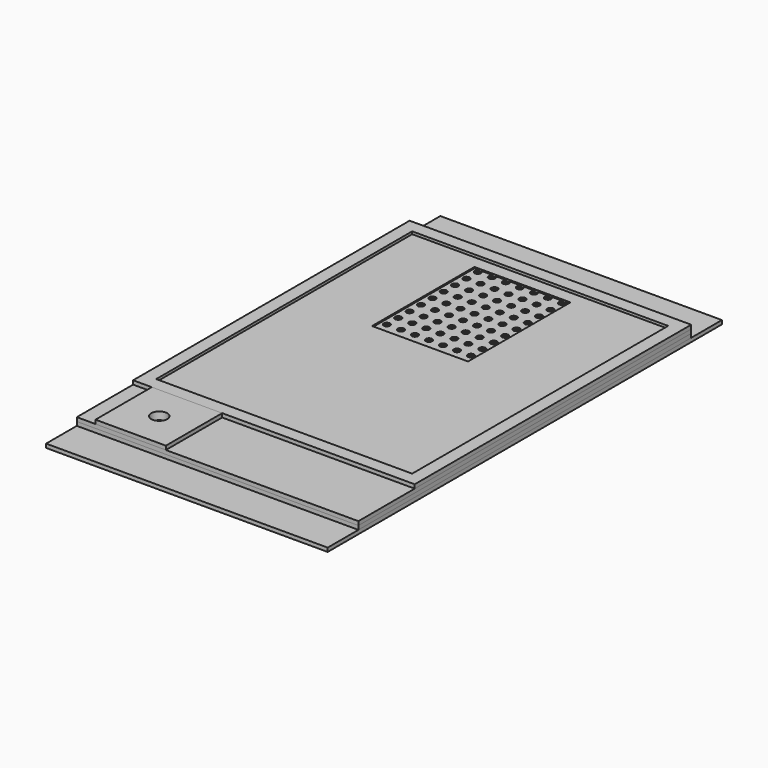
from build123d import *

# Parameters (mm, degrees)
F0_W      = 220
F0_H      = 270
F0_W_2    = 200
F0_H_2    = 250
F1_DEPTH  = 3
F2_W      = 220
F2_H      = 325
F2_R      = 17.07
F2_R_2    = 2.5
F3_DEPTH  = 3
F4_W      = 220
F4_H      = 325
F4_R      = 17.07
F4_R_2    = 1
F5_DEPTH  = 3
F6_W      = 220
F6_H      = 325
F6_W_2    = 90
F6_H_2    = 65
F6_W_3    = 70.7
F6_H_3    = 5.5
F7_DEPTH  = 3
F8_W      = 220
F8_H      = 385
F9_DEPTH  = 3
F10_DEPTH = 3
F11_W     = 55
F11_H     = 55
F12_DEPTH = 3
F13_R     = 6.25
F14_DEPTH = 12.001
F15_W     = 200
F15_H     = 250
F15_W_2   = 75
F15_H_2   = 100
F16_DEPTH = 1
F18_DEPTH = 1


with BuildPart() as f1:
    # F0 (on Top) → F1 (new body)
    with BuildSketch(Plane.XY):
        with Locations((100, 125)):
            Rectangle(F0_W, F0_H)
        with Locations((100, 125)):
            Rectangle(F0_W_2, F0_H_2, mode=Mode.SUBTRACT)
    extrude(amount=F1_DEPTH)


with BuildPart() as f3:
    # F2 (on Top) → F3 (new body)
    with BuildSketch(Plane.XY):
        with Locations((100, 97.5)):
            Rectangle(F2_W, F2_H)
        with Locations((32.07, -37.07)):
            Circle(F2_R, mode=Mode.SUBTRACT)
        with Locations((17.5, 15.5)):
            Circle(F2_R_2, mode=Mode.SUBTRACT)
        with Locations((28.45, 15.5)):
            Circle(F2_R_2, mode=Mode.SUBTRACT)
        with Locations((39.4, 15.5)):
            Circle(F2_R_2, mode=Mode.SUBTRACT)
        with Locations((50.35, 15.5)):
            Circle(F2_R_2, mode=Mode.SUBTRACT)
        with Locations((61.3, 15.5)):
            Circle(F2_R_2, mode=Mode.SUBTRACT)
        with Locations((72.25, 15.5)):
            Circle(F2_R_2, mode=Mode.SUBTRACT)
        with Locations((83.2, 15.5)):
            Circle(F2_R_2, mode=Mode.SUBTRACT)
        with Locations((94.15, 15.5)):
            Circle(F2_R_2, mode=Mode.SUBTRACT)
        with Locations((17.5, 26.6)):
            Circle(F2_R_2, mode=Mode.SUBTRACT)
        with Locations((28.45, 26.6)):
            Circle(F2_R_2, mode=Mode.SUBTRACT)
        with Locations((39.4, 26.6)):
            Circle(F2_R_2, mode=Mode.SUBTRACT)
        with Locations((17.5, 37.7)):
            Circle(F2_R_2, mode=Mode.SUBTRACT)
        with Locations((28.45, 37.7)):
            Circle(F2_R_2, mode=Mode.SUBTRACT)
        with Locations((17.5, 48.8)):
            Circle(F2_R_2, mode=Mode.SUBTRACT)
        with Locations((28.45, 48.8)):
            Circle(F2_R_2, mode=Mode.SUBTRACT)
        with Locations((39.4, 37.7)):
            Circle(F2_R_2, mode=Mode.SUBTRACT)
        with Locations((39.4, 48.8)):
            Circle(F2_R_2, mode=Mode.SUBTRACT)
        with Locations((17.5, 59.9)):
            Circle(F2_R_2, mode=Mode.SUBTRACT)
        with Locations((28.45, 59.9)):
            Circle(F2_R_2, mode=Mode.SUBTRACT)
        with Locations((17.5, 71)):
            Circle(F2_R_2, mode=Mode.SUBTRACT)
        with Locations((28.45, 71)):
            Circle(F2_R_2, mode=Mode.SUBTRACT)
        with Locations((39.4, 59.9)):
            Circle(F2_R_2, mode=Mode.SUBTRACT)
        with Locations((39.4, 71)):
            Circle(F2_R_2, mode=Mode.SUBTRACT)
        with Locations((17.5, 82.1)):
            Circle(F2_R_2, mode=Mode.SUBTRACT)
        with Locations((28.45, 82.1)):
            Circle(F2_R_2, mode=Mode.SUBTRACT)
        with Locations((17.5, 93.2)):
            Circle(F2_R_2, mode=Mode.SUBTRACT)
        with Locations((28.45, 93.2)):
            Circle(F2_R_2, mode=Mode.SUBTRACT)
        with Locations((39.4, 82.1)):
            Circle(F2_R_2, mode=Mode.SUBTRACT)
        with Locations((39.4, 93.2)):
            Circle(F2_R_2, mode=Mode.SUBTRACT)
        with Locations((50.35, 26.6)):
            Circle(F2_R_2, mode=Mode.SUBTRACT)
        with Locations((61.3, 26.6)):
            Circle(F2_R_2, mode=Mode.SUBTRACT)
        with Locations((72.25, 26.6)):
            Circle(F2_R_2, mode=Mode.SUBTRACT)
        with Locations((50.35, 37.7)):
            Circle(F2_R_2, mode=Mode.SUBTRACT)
        with Locations((50.35, 48.8)):
            Circle(F2_R_2, mode=Mode.SUBTRACT)
        with Locations((61.3, 37.7)):
            Circle(F2_R_2, mode=Mode.SUBTRACT)
        with Locations((72.25, 37.7)):
            Circle(F2_R_2, mode=Mode.SUBTRACT)
        with Locations((61.3, 48.8)):
            Circle(F2_R_2, mode=Mode.SUBTRACT)
        with Locations((72.25, 48.8)):
            Circle(F2_R_2, mode=Mode.SUBTRACT)
        with Locations((83.2, 26.6)):
            Circle(F2_R_2, mode=Mode.SUBTRACT)
        with Locations((94.15, 26.6)):
            Circle(F2_R_2, mode=Mode.SUBTRACT)
        with Locations((83.2, 37.7)):
            Circle(F2_R_2, mode=Mode.SUBTRACT)
        with Locations((83.2, 48.8)):
            Circle(F2_R_2, mode=Mode.SUBTRACT)
        with Locations((94.15, 37.7)):
            Circle(F2_R_2, mode=Mode.SUBTRACT)
        with Locations((94.15, 48.8)):
            Circle(F2_R_2, mode=Mode.SUBTRACT)
        with Locations((50.35, 59.9)):
            Circle(F2_R_2, mode=Mode.SUBTRACT)
        with Locations((50.35, 71)):
            Circle(F2_R_2, mode=Mode.SUBTRACT)
        with Locations((61.3, 59.9)):
            Circle(F2_R_2, mode=Mode.SUBTRACT)
        with Locations((72.25, 59.9)):
            Circle(F2_R_2, mode=Mode.SUBTRACT)
        with Locations((61.3, 71)):
            Circle(F2_R_2, mode=Mode.SUBTRACT)
        with Locations((72.25, 71)):
            Circle(F2_R_2, mode=Mode.SUBTRACT)
        with Locations((50.35, 82.1)):
            Circle(F2_R_2, mode=Mode.SUBTRACT)
        with Locations((50.35, 93.2)):
            Circle(F2_R_2, mode=Mode.SUBTRACT)
        with Locations((61.3, 82.1)):
            Circle(F2_R_2, mode=Mode.SUBTRACT)
        with Locations((72.25, 82.1)):
            Circle(F2_R_2, mode=Mode.SUBTRACT)
        with Locations((61.3, 93.2)):
            Circle(F2_R_2, mode=Mode.SUBTRACT)
        with Locations((72.25, 93.2)):
            Circle(F2_R_2, mode=Mode.SUBTRACT)
        with Locations((83.2, 59.9)):
            Circle(F2_R_2, mode=Mode.SUBTRACT)
        with Locations((83.2, 71)):
            Circle(F2_R_2, mode=Mode.SUBTRACT)
        with Locations((94.15, 59.9)):
            Circle(F2_R_2, mode=Mode.SUBTRACT)
        with Locations((94.15, 71)):
            Circle(F2_R_2, mode=Mode.SUBTRACT)
        with Locations((83.2, 82.1)):
            Circle(F2_R_2, mode=Mode.SUBTRACT)
        with Locations((83.2, 93.2)):
            Circle(F2_R_2, mode=Mode.SUBTRACT)
        with Locations((94.15, 82.1)):
            Circle(F2_R_2, mode=Mode.SUBTRACT)
        with Locations((94.15, 93.2)):
            Circle(F2_R_2, mode=Mode.SUBTRACT)
        with Locations((105.1, 15.5)):
            Circle(F2_R_2, mode=Mode.SUBTRACT)
        with Locations((116.05, 15.5)):
            Circle(F2_R_2, mode=Mode.SUBTRACT)
        with Locations((127, 15.5)):
            Circle(F2_R_2, mode=Mode.SUBTRACT)
        with Locations((137.95, 15.5)):
            Circle(F2_R_2, mode=Mode.SUBTRACT)
        with Locations((148.9, 15.5)):
            Circle(F2_R_2, mode=Mode.SUBTRACT)
        with Locations((159.85, 15.5)):
            Circle(F2_R_2, mode=Mode.SUBTRACT)
        with Locations((170.8, 15.5)):
            Circle(F2_R_2, mode=Mode.SUBTRACT)
        with Locations((181.75, 15.5)):
            Circle(F2_R_2, mode=Mode.SUBTRACT)
        with Locations((105.1, 26.6)):
            Circle(F2_R_2, mode=Mode.SUBTRACT)
        with Locations((116.05, 26.6)):
            Circle(F2_R_2, mode=Mode.SUBTRACT)
        with Locations((127, 26.6)):
            Circle(F2_R_2, mode=Mode.SUBTRACT)
        with Locations((105.1, 37.7)):
            Circle(F2_R_2, mode=Mode.SUBTRACT)
        with Locations((105.1, 48.8)):
            Circle(F2_R_2, mode=Mode.SUBTRACT)
        with Locations((116.05, 37.7)):
            Circle(F2_R_2, mode=Mode.SUBTRACT)
        with Locations((127, 37.7)):
            Circle(F2_R_2, mode=Mode.SUBTRACT)
        with Locations((116.05, 48.8)):
            Circle(F2_R_2, mode=Mode.SUBTRACT)
        with Locations((127, 48.8)):
            Circle(F2_R_2, mode=Mode.SUBTRACT)
        with Locations((137.95, 26.6)):
            Circle(F2_R_2, mode=Mode.SUBTRACT)
        with Locations((148.9, 26.6)):
            Circle(F2_R_2, mode=Mode.SUBTRACT)
        with Locations((137.95, 37.7)):
            Circle(F2_R_2, mode=Mode.SUBTRACT)
        with Locations((137.95, 48.8)):
            Circle(F2_R_2, mode=Mode.SUBTRACT)
        with Locations((148.9, 37.7)):
            Circle(F2_R_2, mode=Mode.SUBTRACT)
        with Locations((148.9, 48.8)):
            Circle(F2_R_2, mode=Mode.SUBTRACT)
        with Locations((105.1, 59.9)):
            Circle(F2_R_2, mode=Mode.SUBTRACT)
        with Locations((105.1, 71)):
            Circle(F2_R_2, mode=Mode.SUBTRACT)
        with Locations((116.05, 59.9)):
            Circle(F2_R_2, mode=Mode.SUBTRACT)
        with Locations((127, 59.9)):
            Circle(F2_R_2, mode=Mode.SUBTRACT)
        with Locations((116.05, 71)):
            Circle(F2_R_2, mode=Mode.SUBTRACT)
        with Locations((127, 71)):
            Circle(F2_R_2, mode=Mode.SUBTRACT)
        with Locations((105.1, 82.1)):
            Circle(F2_R_2, mode=Mode.SUBTRACT)
        with Locations((105.1, 93.2)):
            Circle(F2_R_2, mode=Mode.SUBTRACT)
        with Locations((116.05, 82.1)):
            Circle(F2_R_2, mode=Mode.SUBTRACT)
        with Locations((127, 82.1)):
            Circle(F2_R_2, mode=Mode.SUBTRACT)
        with Locations((116.05, 93.2)):
            Circle(F2_R_2, mode=Mode.SUBTRACT)
        with Locations((127, 93.2)):
            Circle(F2_R_2, mode=Mode.SUBTRACT)
        with Locations((137.95, 59.9)):
            Circle(F2_R_2, mode=Mode.SUBTRACT)
        with Locations((137.95, 71)):
            Circle(F2_R_2, mode=Mode.SUBTRACT)
        with Locations((148.9, 59.9)):
            Circle(F2_R_2, mode=Mode.SUBTRACT)
        with Locations((148.9, 71)):
            Circle(F2_R_2, mode=Mode.SUBTRACT)
        with Locations((137.95, 82.1)):
            Circle(F2_R_2, mode=Mode.SUBTRACT)
        with Locations((137.95, 93.2)):
            Circle(F2_R_2, mode=Mode.SUBTRACT)
        with Locations((148.9, 82.1)):
            Circle(F2_R_2, mode=Mode.SUBTRACT)
        with Locations((148.9, 93.2)):
            Circle(F2_R_2, mode=Mode.SUBTRACT)
        with Locations((159.85, 26.6)):
            Circle(F2_R_2, mode=Mode.SUBTRACT)
        with Locations((170.8, 26.6)):
            Circle(F2_R_2, mode=Mode.SUBTRACT)
        with Locations((181.75, 26.6)):
            Circle(F2_R_2, mode=Mode.SUBTRACT)
        with Locations((159.85, 37.7)):
            Circle(F2_R_2, mode=Mode.SUBTRACT)
        with Locations((159.85, 48.8)):
            Circle(F2_R_2, mode=Mode.SUBTRACT)
        with Locations((170.8, 37.7)):
            Circle(F2_R_2, mode=Mode.SUBTRACT)
        with Locations((181.75, 37.7)):
            Circle(F2_R_2, mode=Mode.SUBTRACT)
        with Locations((170.8, 48.8)):
            Circle(F2_R_2, mode=Mode.SUBTRACT)
        with Locations((181.75, 48.8)):
            Circle(F2_R_2, mode=Mode.SUBTRACT)
        with Locations((159.85, 59.9)):
            Circle(F2_R_2, mode=Mode.SUBTRACT)
        with Locations((159.85, 71)):
            Circle(F2_R_2, mode=Mode.SUBTRACT)
        with Locations((170.8, 59.9)):
            Circle(F2_R_2, mode=Mode.SUBTRACT)
        with Locations((181.75, 59.9)):
            Circle(F2_R_2, mode=Mode.SUBTRACT)
        with Locations((170.8, 71)):
            Circle(F2_R_2, mode=Mode.SUBTRACT)
        with Locations((181.75, 71)):
            Circle(F2_R_2, mode=Mode.SUBTRACT)
        with Locations((159.85, 82.1)):
            Circle(F2_R_2, mode=Mode.SUBTRACT)
        with Locations((159.85, 93.2)):
            Circle(F2_R_2, mode=Mode.SUBTRACT)
        with Locations((170.8, 82.1)):
            Circle(F2_R_2, mode=Mode.SUBTRACT)
        with Locations((181.75, 82.1)):
            Circle(F2_R_2, mode=Mode.SUBTRACT)
        with Locations((170.8, 93.2)):
            Circle(F2_R_2, mode=Mode.SUBTRACT)
        with Locations((181.75, 93.2)):
            Circle(F2_R_2, mode=Mode.SUBTRACT)
        with Locations((17.5, 104.3)):
            Circle(F2_R_2, mode=Mode.SUBTRACT)
        with Locations((28.45, 104.3)):
            Circle(F2_R_2, mode=Mode.SUBTRACT)
        with Locations((17.5, 115.4)):
            Circle(F2_R_2, mode=Mode.SUBTRACT)
        with Locations((28.45, 115.4)):
            Circle(F2_R_2, mode=Mode.SUBTRACT)
        with Locations((39.4, 104.3)):
            Circle(F2_R_2, mode=Mode.SUBTRACT)
        with Locations((39.4, 115.4)):
            Circle(F2_R_2, mode=Mode.SUBTRACT)
        with Locations((17.5, 126.5)):
            Circle(F2_R_2, mode=Mode.SUBTRACT)
        with Locations((28.45, 126.5)):
            Circle(F2_R_2, mode=Mode.SUBTRACT)
        with Locations((17.5, 137.6)):
            Circle(F2_R_2, mode=Mode.SUBTRACT)
        with Locations((28.45, 137.6)):
            Circle(F2_R_2, mode=Mode.SUBTRACT)
        with Locations((39.4, 126.5)):
            Circle(F2_R_2, mode=Mode.SUBTRACT)
        with Locations((39.4, 137.6)):
            Circle(F2_R_2, mode=Mode.SUBTRACT)
        with Locations((17.5, 148.7)):
            Circle(F2_R_2, mode=Mode.SUBTRACT)
        with Locations((28.45, 148.7)):
            Circle(F2_R_2, mode=Mode.SUBTRACT)
        with Locations((39.4, 148.7)):
            Circle(F2_R_2, mode=Mode.SUBTRACT)
        with Locations((17.5, 159.8)):
            Circle(F2_R_2, mode=Mode.SUBTRACT)
        with Locations((28.45, 159.8)):
            Circle(F2_R_2, mode=Mode.SUBTRACT)
        with Locations((17.5, 170.9)):
            Circle(F2_R_2, mode=Mode.SUBTRACT)
        with Locations((28.45, 170.9)):
            Circle(F2_R_2, mode=Mode.SUBTRACT)
        with Locations((39.4, 159.8)):
            Circle(F2_R_2, mode=Mode.SUBTRACT)
        with Locations((39.4, 170.9)):
            Circle(F2_R_2, mode=Mode.SUBTRACT)
        with Locations((50.35, 104.3)):
            Circle(F2_R_2, mode=Mode.SUBTRACT)
        with Locations((50.35, 115.4)):
            Circle(F2_R_2, mode=Mode.SUBTRACT)
        with Locations((61.3, 104.3)):
            Circle(F2_R_2, mode=Mode.SUBTRACT)
        with Locations((72.25, 104.3)):
            Circle(F2_R_2, mode=Mode.SUBTRACT)
        with Locations((61.3, 115.4)):
            Circle(F2_R_2, mode=Mode.SUBTRACT)
        with Locations((72.25, 115.4)):
            Circle(F2_R_2, mode=Mode.SUBTRACT)
        with Locations((50.35, 126.5)):
            Circle(F2_R_2, mode=Mode.SUBTRACT)
        with Locations((50.35, 137.6)):
            Circle(F2_R_2, mode=Mode.SUBTRACT)
        with Locations((61.3, 126.5)):
            Circle(F2_R_2, mode=Mode.SUBTRACT)
        with Locations((72.25, 126.5)):
            Circle(F2_R_2, mode=Mode.SUBTRACT)
        with Locations((61.3, 137.6)):
            Circle(F2_R_2, mode=Mode.SUBTRACT)
        with Locations((72.25, 137.6)):
            Circle(F2_R_2, mode=Mode.SUBTRACT)
        with Locations((83.2, 104.3)):
            Circle(F2_R_2, mode=Mode.SUBTRACT)
        with Locations((83.2, 115.4)):
            Circle(F2_R_2, mode=Mode.SUBTRACT)
        with Locations((94.15, 104.3)):
            Circle(F2_R_2, mode=Mode.SUBTRACT)
        with Locations((94.15, 115.4)):
            Circle(F2_R_2, mode=Mode.SUBTRACT)
        with Locations((83.2, 126.5)):
            Circle(F2_R_2, mode=Mode.SUBTRACT)
        with Locations((83.2, 137.6)):
            Circle(F2_R_2, mode=Mode.SUBTRACT)
        with Locations((94.15, 126.5)):
            Circle(F2_R_2, mode=Mode.SUBTRACT)
        with Locations((94.15, 137.6)):
            Circle(F2_R_2, mode=Mode.SUBTRACT)
        with Locations((50.35, 148.7)):
            Circle(F2_R_2, mode=Mode.SUBTRACT)
        with Locations((61.3, 148.7)):
            Circle(F2_R_2, mode=Mode.SUBTRACT)
        with Locations((72.25, 148.7)):
            Circle(F2_R_2, mode=Mode.SUBTRACT)
        with Locations((50.35, 159.8)):
            Circle(F2_R_2, mode=Mode.SUBTRACT)
        with Locations((50.35, 170.9)):
            Circle(F2_R_2, mode=Mode.SUBTRACT)
        with Locations((61.3, 159.8)):
            Circle(F2_R_2, mode=Mode.SUBTRACT)
        with Locations((72.25, 159.8)):
            Circle(F2_R_2, mode=Mode.SUBTRACT)
        with Locations((61.3, 170.9)):
            Circle(F2_R_2, mode=Mode.SUBTRACT)
        with Locations((72.25, 170.9)):
            Circle(F2_R_2, mode=Mode.SUBTRACT)
        with Locations((83.2, 148.7)):
            Circle(F2_R_2, mode=Mode.SUBTRACT)
        with Locations((94.15, 148.7)):
            Circle(F2_R_2, mode=Mode.SUBTRACT)
        with Locations((83.2, 159.8)):
            Circle(F2_R_2, mode=Mode.SUBTRACT)
        with Locations((83.2, 170.9)):
            Circle(F2_R_2, mode=Mode.SUBTRACT)
        with Locations((94.15, 159.8)):
            Circle(F2_R_2, mode=Mode.SUBTRACT)
        with Locations((94.15, 170.9)):
            Circle(F2_R_2, mode=Mode.SUBTRACT)
        with Locations((17.5, 182)):
            Circle(F2_R_2, mode=Mode.SUBTRACT)
        with Locations((28.45, 182)):
            Circle(F2_R_2, mode=Mode.SUBTRACT)
        with Locations((17.5, 193.1)):
            Circle(F2_R_2, mode=Mode.SUBTRACT)
        with Locations((28.45, 193.1)):
            Circle(F2_R_2, mode=Mode.SUBTRACT)
        with Locations((39.4, 182)):
            Circle(F2_R_2, mode=Mode.SUBTRACT)
        with Locations((39.4, 193.1)):
            Circle(F2_R_2, mode=Mode.SUBTRACT)
        with Locations((17.5, 204.2)):
            Circle(F2_R_2, mode=Mode.SUBTRACT)
        with Locations((28.45, 204.2)):
            Circle(F2_R_2, mode=Mode.SUBTRACT)
        with Locations((17.5, 215.3)):
            Circle(F2_R_2, mode=Mode.SUBTRACT)
        with Locations((28.45, 215.3)):
            Circle(F2_R_2, mode=Mode.SUBTRACT)
        with Locations((39.4, 204.2)):
            Circle(F2_R_2, mode=Mode.SUBTRACT)
        with Locations((39.4, 215.3)):
            Circle(F2_R_2, mode=Mode.SUBTRACT)
        with Locations((17.5, 226.4)):
            Circle(F2_R_2, mode=Mode.SUBTRACT)
        with Locations((28.45, 226.4)):
            Circle(F2_R_2, mode=Mode.SUBTRACT)
        with Locations((17.5, 237.5)):
            Circle(F2_R_2, mode=Mode.SUBTRACT)
        with Locations((28.45, 237.5)):
            Circle(F2_R_2, mode=Mode.SUBTRACT)
        with Locations((39.4, 226.4)):
            Circle(F2_R_2, mode=Mode.SUBTRACT)
        with Locations((39.4, 237.5)):
            Circle(F2_R_2, mode=Mode.SUBTRACT)
        with Locations((50.35, 182)):
            Circle(F2_R_2, mode=Mode.SUBTRACT)
        with Locations((50.35, 193.1)):
            Circle(F2_R_2, mode=Mode.SUBTRACT)
        with Locations((61.3, 182)):
            Circle(F2_R_2, mode=Mode.SUBTRACT)
        with Locations((72.25, 182)):
            Circle(F2_R_2, mode=Mode.SUBTRACT)
        with Locations((61.3, 193.1)):
            Circle(F2_R_2, mode=Mode.SUBTRACT)
        with Locations((72.25, 193.1)):
            Circle(F2_R_2, mode=Mode.SUBTRACT)
        with Locations((50.35, 204.2)):
            Circle(F2_R_2, mode=Mode.SUBTRACT)
        with Locations((50.35, 215.3)):
            Circle(F2_R_2, mode=Mode.SUBTRACT)
        with Locations((61.3, 204.2)):
            Circle(F2_R_2, mode=Mode.SUBTRACT)
        with Locations((72.25, 204.2)):
            Circle(F2_R_2, mode=Mode.SUBTRACT)
        with Locations((61.3, 215.3)):
            Circle(F2_R_2, mode=Mode.SUBTRACT)
        with Locations((72.25, 215.3)):
            Circle(F2_R_2, mode=Mode.SUBTRACT)
        with Locations((83.2, 182)):
            Circle(F2_R_2, mode=Mode.SUBTRACT)
        with Locations((83.2, 193.1)):
            Circle(F2_R_2, mode=Mode.SUBTRACT)
        with Locations((94.15, 182)):
            Circle(F2_R_2, mode=Mode.SUBTRACT)
        with Locations((94.15, 193.1)):
            Circle(F2_R_2, mode=Mode.SUBTRACT)
        with Locations((83.2, 204.2)):
            Circle(F2_R_2, mode=Mode.SUBTRACT)
        with Locations((83.2, 215.3)):
            Circle(F2_R_2, mode=Mode.SUBTRACT)
        with Locations((94.15, 204.2)):
            Circle(F2_R_2, mode=Mode.SUBTRACT)
        with Locations((94.15, 215.3)):
            Circle(F2_R_2, mode=Mode.SUBTRACT)
        with Locations((50.35, 226.4)):
            Circle(F2_R_2, mode=Mode.SUBTRACT)
        with Locations((50.35, 237.5)):
            Circle(F2_R_2, mode=Mode.SUBTRACT)
        with Locations((61.3, 226.4)):
            Circle(F2_R_2, mode=Mode.SUBTRACT)
        with Locations((72.25, 226.4)):
            Circle(F2_R_2, mode=Mode.SUBTRACT)
        with Locations((61.3, 237.5)):
            Circle(F2_R_2, mode=Mode.SUBTRACT)
        with Locations((72.25, 237.5)):
            Circle(F2_R_2, mode=Mode.SUBTRACT)
        with Locations((83.2, 226.4)):
            Circle(F2_R_2, mode=Mode.SUBTRACT)
        with Locations((83.2, 237.5)):
            Circle(F2_R_2, mode=Mode.SUBTRACT)
        with Locations((94.15, 226.4)):
            Circle(F2_R_2, mode=Mode.SUBTRACT)
        with Locations((94.15, 237.5)):
            Circle(F2_R_2, mode=Mode.SUBTRACT)
        with Locations((105.1, 104.3)):
            Circle(F2_R_2, mode=Mode.SUBTRACT)
        with Locations((105.1, 115.4)):
            Circle(F2_R_2, mode=Mode.SUBTRACT)
        with Locations((116.05, 104.3)):
            Circle(F2_R_2, mode=Mode.SUBTRACT)
        with Locations((127, 104.3)):
            Circle(F2_R_2, mode=Mode.SUBTRACT)
        with Locations((116.05, 115.4)):
            Circle(F2_R_2, mode=Mode.SUBTRACT)
        with Locations((127, 115.4)):
            Circle(F2_R_2, mode=Mode.SUBTRACT)
        with Locations((105.1, 126.5)):
            Circle(F2_R_2, mode=Mode.SUBTRACT)
        with Locations((105.1, 137.6)):
            Circle(F2_R_2, mode=Mode.SUBTRACT)
        with Locations((116.05, 126.5)):
            Circle(F2_R_2, mode=Mode.SUBTRACT)
        with Locations((127, 126.5)):
            Circle(F2_R_2, mode=Mode.SUBTRACT)
        with Locations((116.05, 137.6)):
            Circle(F2_R_2, mode=Mode.SUBTRACT)
        with Locations((127, 137.6)):
            Circle(F2_R_2, mode=Mode.SUBTRACT)
        with Locations((137.95, 104.3)):
            Circle(F2_R_2, mode=Mode.SUBTRACT)
        with Locations((137.95, 115.4)):
            Circle(F2_R_2, mode=Mode.SUBTRACT)
        with Locations((148.9, 104.3)):
            Circle(F2_R_2, mode=Mode.SUBTRACT)
        with Locations((148.9, 115.4)):
            Circle(F2_R_2, mode=Mode.SUBTRACT)
        with Locations((137.95, 126.5)):
            Circle(F2_R_2, mode=Mode.SUBTRACT)
        with Locations((137.95, 137.6)):
            Circle(F2_R_2, mode=Mode.SUBTRACT)
        with Locations((148.9, 126.5)):
            Circle(F2_R_2, mode=Mode.SUBTRACT)
        with Locations((148.9, 137.6)):
            Circle(F2_R_2, mode=Mode.SUBTRACT)
        with Locations((105.1, 148.7)):
            Circle(F2_R_2, mode=Mode.SUBTRACT)
        with Locations((116.05, 148.7)):
            Circle(F2_R_2, mode=Mode.SUBTRACT)
        with Locations((127, 148.7)):
            Circle(F2_R_2, mode=Mode.SUBTRACT)
        with Locations((105.1, 159.8)):
            Circle(F2_R_2, mode=Mode.SUBTRACT)
        with Locations((105.1, 170.9)):
            Circle(F2_R_2, mode=Mode.SUBTRACT)
        with Locations((116.05, 159.8)):
            Circle(F2_R_2, mode=Mode.SUBTRACT)
        with Locations((127, 159.8)):
            Circle(F2_R_2, mode=Mode.SUBTRACT)
        with Locations((116.05, 170.9)):
            Circle(F2_R_2, mode=Mode.SUBTRACT)
        with Locations((127, 170.9)):
            Circle(F2_R_2, mode=Mode.SUBTRACT)
        with Locations((137.95, 148.7)):
            Circle(F2_R_2, mode=Mode.SUBTRACT)
        with Locations((148.9, 148.7)):
            Circle(F2_R_2, mode=Mode.SUBTRACT)
        with Locations((137.95, 159.8)):
            Circle(F2_R_2, mode=Mode.SUBTRACT)
        with Locations((137.95, 170.9)):
            Circle(F2_R_2, mode=Mode.SUBTRACT)
        with Locations((148.9, 159.8)):
            Circle(F2_R_2, mode=Mode.SUBTRACT)
        with Locations((148.9, 170.9)):
            Circle(F2_R_2, mode=Mode.SUBTRACT)
        with Locations((159.85, 104.3)):
            Circle(F2_R_2, mode=Mode.SUBTRACT)
        with Locations((159.85, 115.4)):
            Circle(F2_R_2, mode=Mode.SUBTRACT)
        with Locations((170.8, 104.3)):
            Circle(F2_R_2, mode=Mode.SUBTRACT)
        with Locations((181.75, 104.3)):
            Circle(F2_R_2, mode=Mode.SUBTRACT)
        with Locations((170.8, 115.4)):
            Circle(F2_R_2, mode=Mode.SUBTRACT)
        with Locations((181.75, 115.4)):
            Circle(F2_R_2, mode=Mode.SUBTRACT)
        with Locations((159.85, 126.5)):
            Circle(F2_R_2, mode=Mode.SUBTRACT)
        with Locations((159.85, 137.6)):
            Circle(F2_R_2, mode=Mode.SUBTRACT)
        with Locations((170.8, 126.5)):
            Circle(F2_R_2, mode=Mode.SUBTRACT)
        with Locations((181.75, 126.5)):
            Circle(F2_R_2, mode=Mode.SUBTRACT)
        with Locations((170.8, 137.6)):
            Circle(F2_R_2, mode=Mode.SUBTRACT)
        with Locations((181.75, 137.6)):
            Circle(F2_R_2, mode=Mode.SUBTRACT)
        with Locations((159.85, 148.7)):
            Circle(F2_R_2, mode=Mode.SUBTRACT)
        with Locations((170.8, 148.7)):
            Circle(F2_R_2, mode=Mode.SUBTRACT)
        with Locations((181.75, 148.7)):
            Circle(F2_R_2, mode=Mode.SUBTRACT)
        with Locations((159.85, 159.8)):
            Circle(F2_R_2, mode=Mode.SUBTRACT)
        with Locations((159.85, 170.9)):
            Circle(F2_R_2, mode=Mode.SUBTRACT)
        with Locations((170.8, 159.8)):
            Circle(F2_R_2, mode=Mode.SUBTRACT)
        with Locations((181.75, 159.8)):
            Circle(F2_R_2, mode=Mode.SUBTRACT)
        with Locations((170.8, 170.9)):
            Circle(F2_R_2, mode=Mode.SUBTRACT)
        with Locations((181.75, 170.9)):
            Circle(F2_R_2, mode=Mode.SUBTRACT)
        with Locations((105.1, 182)):
            Circle(F2_R_2, mode=Mode.SUBTRACT)
        with Locations((105.1, 193.1)):
            Circle(F2_R_2, mode=Mode.SUBTRACT)
        with Locations((116.05, 182)):
            Circle(F2_R_2, mode=Mode.SUBTRACT)
        with Locations((127, 182)):
            Circle(F2_R_2, mode=Mode.SUBTRACT)
        with Locations((116.05, 193.1)):
            Circle(F2_R_2, mode=Mode.SUBTRACT)
        with Locations((127, 193.1)):
            Circle(F2_R_2, mode=Mode.SUBTRACT)
        with Locations((105.1, 204.2)):
            Circle(F2_R_2, mode=Mode.SUBTRACT)
        with Locations((105.1, 215.3)):
            Circle(F2_R_2, mode=Mode.SUBTRACT)
        with Locations((116.05, 204.2)):
            Circle(F2_R_2, mode=Mode.SUBTRACT)
        with Locations((127, 204.2)):
            Circle(F2_R_2, mode=Mode.SUBTRACT)
        with Locations((116.05, 215.3)):
            Circle(F2_R_2, mode=Mode.SUBTRACT)
        with Locations((127, 215.3)):
            Circle(F2_R_2, mode=Mode.SUBTRACT)
        with Locations((137.95, 182)):
            Circle(F2_R_2, mode=Mode.SUBTRACT)
        with Locations((137.95, 193.1)):
            Circle(F2_R_2, mode=Mode.SUBTRACT)
        with Locations((148.9, 182)):
            Circle(F2_R_2, mode=Mode.SUBTRACT)
        with Locations((148.9, 193.1)):
            Circle(F2_R_2, mode=Mode.SUBTRACT)
        with Locations((137.95, 204.2)):
            Circle(F2_R_2, mode=Mode.SUBTRACT)
        with Locations((137.95, 215.3)):
            Circle(F2_R_2, mode=Mode.SUBTRACT)
        with Locations((148.9, 204.2)):
            Circle(F2_R_2, mode=Mode.SUBTRACT)
        with Locations((148.9, 215.3)):
            Circle(F2_R_2, mode=Mode.SUBTRACT)
        with Locations((105.1, 226.4)):
            Circle(F2_R_2, mode=Mode.SUBTRACT)
        with Locations((105.1, 237.5)):
            Circle(F2_R_2, mode=Mode.SUBTRACT)
        with Locations((116.05, 226.4)):
            Circle(F2_R_2, mode=Mode.SUBTRACT)
        with Locations((127, 226.4)):
            Circle(F2_R_2, mode=Mode.SUBTRACT)
        with Locations((116.05, 237.5)):
            Circle(F2_R_2, mode=Mode.SUBTRACT)
        with Locations((127, 237.5)):
            Circle(F2_R_2, mode=Mode.SUBTRACT)
        with Locations((137.95, 226.4)):
            Circle(F2_R_2, mode=Mode.SUBTRACT)
        with Locations((137.95, 237.5)):
            Circle(F2_R_2, mode=Mode.SUBTRACT)
        with Locations((148.9, 226.4)):
            Circle(F2_R_2, mode=Mode.SUBTRACT)
        with Locations((148.9, 237.5)):
            Circle(F2_R_2, mode=Mode.SUBTRACT)
        with Locations((159.85, 182)):
            Circle(F2_R_2, mode=Mode.SUBTRACT)
        with Locations((159.85, 193.1)):
            Circle(F2_R_2, mode=Mode.SUBTRACT)
        with Locations((170.8, 182)):
            Circle(F2_R_2, mode=Mode.SUBTRACT)
        with Locations((181.75, 182)):
            Circle(F2_R_2, mode=Mode.SUBTRACT)
        with Locations((170.8, 193.1)):
            Circle(F2_R_2, mode=Mode.SUBTRACT)
        with Locations((181.75, 193.1)):
            Circle(F2_R_2, mode=Mode.SUBTRACT)
        with Locations((159.85, 204.2)):
            Circle(F2_R_2, mode=Mode.SUBTRACT)
        with Locations((159.85, 215.3)):
            Circle(F2_R_2, mode=Mode.SUBTRACT)
        with Locations((170.8, 204.2)):
            Circle(F2_R_2, mode=Mode.SUBTRACT)
        with Locations((181.75, 204.2)):
            Circle(F2_R_2, mode=Mode.SUBTRACT)
        with Locations((170.8, 215.3)):
            Circle(F2_R_2, mode=Mode.SUBTRACT)
        with Locations((181.75, 215.3)):
            Circle(F2_R_2, mode=Mode.SUBTRACT)
        with Locations((159.85, 226.4)):
            Circle(F2_R_2, mode=Mode.SUBTRACT)
        with Locations((159.85, 237.5)):
            Circle(F2_R_2, mode=Mode.SUBTRACT)
        with Locations((170.8, 226.4)):
            Circle(F2_R_2, mode=Mode.SUBTRACT)
        with Locations((181.75, 226.4)):
            Circle(F2_R_2, mode=Mode.SUBTRACT)
        with Locations((170.8, 237.5)):
            Circle(F2_R_2, mode=Mode.SUBTRACT)
        with Locations((181.75, 237.5)):
            Circle(F2_R_2, mode=Mode.SUBTRACT)
    extrude(amount=-F3_DEPTH)


with BuildPart() as f5:
    # F4 (on Top) → F5 (new body)
    with BuildSketch(Plane.XY):
        with Locations((100, 97.5)):
            Rectangle(F4_W, F4_H)
        with Locations((32.07, -37.07)):
            Circle(F4_R, mode=Mode.SUBTRACT)
        with Locations((17.5, 15.5)):
            Circle(F4_R_2, mode=Mode.SUBTRACT)
        with Locations((28.45, 15.5)):
            Circle(F4_R_2, mode=Mode.SUBTRACT)
        with Locations((39.4, 15.5)):
            Circle(F4_R_2, mode=Mode.SUBTRACT)
        with Locations((50.35, 15.5)):
            Circle(F4_R_2, mode=Mode.SUBTRACT)
        with Locations((61.3, 15.5)):
            Circle(F4_R_2, mode=Mode.SUBTRACT)
        with Locations((72.25, 15.5)):
            Circle(F4_R_2, mode=Mode.SUBTRACT)
        with Locations((83.2, 15.5)):
            Circle(F4_R_2, mode=Mode.SUBTRACT)
        with Locations((94.15, 15.5)):
            Circle(F4_R_2, mode=Mode.SUBTRACT)
        with Locations((17.5, 26.6)):
            Circle(F4_R_2, mode=Mode.SUBTRACT)
        with Locations((28.45, 26.6)):
            Circle(F4_R_2, mode=Mode.SUBTRACT)
        with Locations((39.4, 26.6)):
            Circle(F4_R_2, mode=Mode.SUBTRACT)
        with Locations((17.5, 37.7)):
            Circle(F4_R_2, mode=Mode.SUBTRACT)
        with Locations((28.45, 37.7)):
            Circle(F4_R_2, mode=Mode.SUBTRACT)
        with Locations((17.5, 48.8)):
            Circle(F4_R_2, mode=Mode.SUBTRACT)
        with Locations((28.45, 48.8)):
            Circle(F4_R_2, mode=Mode.SUBTRACT)
        with Locations((39.4, 37.7)):
            Circle(F4_R_2, mode=Mode.SUBTRACT)
        with Locations((39.4, 48.8)):
            Circle(F4_R_2, mode=Mode.SUBTRACT)
        with Locations((17.5, 59.9)):
            Circle(F4_R_2, mode=Mode.SUBTRACT)
        with Locations((28.45, 59.9)):
            Circle(F4_R_2, mode=Mode.SUBTRACT)
        with Locations((17.5, 71)):
            Circle(F4_R_2, mode=Mode.SUBTRACT)
        with Locations((28.45, 71)):
            Circle(F4_R_2, mode=Mode.SUBTRACT)
        with Locations((39.4, 59.9)):
            Circle(F4_R_2, mode=Mode.SUBTRACT)
        with Locations((39.4, 71)):
            Circle(F4_R_2, mode=Mode.SUBTRACT)
        with Locations((17.5, 82.1)):
            Circle(F4_R_2, mode=Mode.SUBTRACT)
        with Locations((28.45, 82.1)):
            Circle(F4_R_2, mode=Mode.SUBTRACT)
        with Locations((17.5, 93.2)):
            Circle(F4_R_2, mode=Mode.SUBTRACT)
        with Locations((28.45, 93.2)):
            Circle(F4_R_2, mode=Mode.SUBTRACT)
        with Locations((39.4, 82.1)):
            Circle(F4_R_2, mode=Mode.SUBTRACT)
        with Locations((39.4, 93.2)):
            Circle(F4_R_2, mode=Mode.SUBTRACT)
        with Locations((50.35, 26.6)):
            Circle(F4_R_2, mode=Mode.SUBTRACT)
        with Locations((61.3, 26.6)):
            Circle(F4_R_2, mode=Mode.SUBTRACT)
        with Locations((72.25, 26.6)):
            Circle(F4_R_2, mode=Mode.SUBTRACT)
        with Locations((50.35, 37.7)):
            Circle(F4_R_2, mode=Mode.SUBTRACT)
        with Locations((50.35, 48.8)):
            Circle(F4_R_2, mode=Mode.SUBTRACT)
        with Locations((61.3, 37.7)):
            Circle(F4_R_2, mode=Mode.SUBTRACT)
        with Locations((72.25, 37.7)):
            Circle(F4_R_2, mode=Mode.SUBTRACT)
        with Locations((61.3, 48.8)):
            Circle(F4_R_2, mode=Mode.SUBTRACT)
        with Locations((72.25, 48.8)):
            Circle(F4_R_2, mode=Mode.SUBTRACT)
        with Locations((83.2, 26.6)):
            Circle(F4_R_2, mode=Mode.SUBTRACT)
        with Locations((94.15, 26.6)):
            Circle(F4_R_2, mode=Mode.SUBTRACT)
        with Locations((83.2, 37.7)):
            Circle(F4_R_2, mode=Mode.SUBTRACT)
        with Locations((83.2, 48.8)):
            Circle(F4_R_2, mode=Mode.SUBTRACT)
        with Locations((94.15, 37.7)):
            Circle(F4_R_2, mode=Mode.SUBTRACT)
        with Locations((94.15, 48.8)):
            Circle(F4_R_2, mode=Mode.SUBTRACT)
        with Locations((50.35, 59.9)):
            Circle(F4_R_2, mode=Mode.SUBTRACT)
        with Locations((50.35, 71)):
            Circle(F4_R_2, mode=Mode.SUBTRACT)
        with Locations((61.3, 59.9)):
            Circle(F4_R_2, mode=Mode.SUBTRACT)
        with Locations((72.25, 59.9)):
            Circle(F4_R_2, mode=Mode.SUBTRACT)
        with Locations((61.3, 71)):
            Circle(F4_R_2, mode=Mode.SUBTRACT)
        with Locations((72.25, 71)):
            Circle(F4_R_2, mode=Mode.SUBTRACT)
        with Locations((50.35, 82.1)):
            Circle(F4_R_2, mode=Mode.SUBTRACT)
        with Locations((50.35, 93.2)):
            Circle(F4_R_2, mode=Mode.SUBTRACT)
        with Locations((61.3, 82.1)):
            Circle(F4_R_2, mode=Mode.SUBTRACT)
        with Locations((72.25, 82.1)):
            Circle(F4_R_2, mode=Mode.SUBTRACT)
        with Locations((61.3, 93.2)):
            Circle(F4_R_2, mode=Mode.SUBTRACT)
        with Locations((72.25, 93.2)):
            Circle(F4_R_2, mode=Mode.SUBTRACT)
        with Locations((83.2, 59.9)):
            Circle(F4_R_2, mode=Mode.SUBTRACT)
        with Locations((83.2, 71)):
            Circle(F4_R_2, mode=Mode.SUBTRACT)
        with Locations((94.15, 59.9)):
            Circle(F4_R_2, mode=Mode.SUBTRACT)
        with Locations((94.15, 71)):
            Circle(F4_R_2, mode=Mode.SUBTRACT)
        with Locations((83.2, 82.1)):
            Circle(F4_R_2, mode=Mode.SUBTRACT)
        with Locations((83.2, 93.2)):
            Circle(F4_R_2, mode=Mode.SUBTRACT)
        with Locations((94.15, 82.1)):
            Circle(F4_R_2, mode=Mode.SUBTRACT)
        with Locations((94.15, 93.2)):
            Circle(F4_R_2, mode=Mode.SUBTRACT)
        with Locations((105.1, 15.5)):
            Circle(F4_R_2, mode=Mode.SUBTRACT)
        with Locations((116.05, 15.5)):
            Circle(F4_R_2, mode=Mode.SUBTRACT)
        with Locations((127, 15.5)):
            Circle(F4_R_2, mode=Mode.SUBTRACT)
        with Locations((137.95, 15.5)):
            Circle(F4_R_2, mode=Mode.SUBTRACT)
        with Locations((148.9, 15.5)):
            Circle(F4_R_2, mode=Mode.SUBTRACT)
        with Locations((159.85, 15.5)):
            Circle(F4_R_2, mode=Mode.SUBTRACT)
        with Locations((170.8, 15.5)):
            Circle(F4_R_2, mode=Mode.SUBTRACT)
        with Locations((181.75, 15.5)):
            Circle(F4_R_2, mode=Mode.SUBTRACT)
        with Locations((105.1, 26.6)):
            Circle(F4_R_2, mode=Mode.SUBTRACT)
        with Locations((116.05, 26.6)):
            Circle(F4_R_2, mode=Mode.SUBTRACT)
        with Locations((127, 26.6)):
            Circle(F4_R_2, mode=Mode.SUBTRACT)
        with Locations((105.1, 37.7)):
            Circle(F4_R_2, mode=Mode.SUBTRACT)
        with Locations((105.1, 48.8)):
            Circle(F4_R_2, mode=Mode.SUBTRACT)
        with Locations((116.05, 37.7)):
            Circle(F4_R_2, mode=Mode.SUBTRACT)
        with Locations((127, 37.7)):
            Circle(F4_R_2, mode=Mode.SUBTRACT)
        with Locations((116.05, 48.8)):
            Circle(F4_R_2, mode=Mode.SUBTRACT)
        with Locations((127, 48.8)):
            Circle(F4_R_2, mode=Mode.SUBTRACT)
        with Locations((137.95, 26.6)):
            Circle(F4_R_2, mode=Mode.SUBTRACT)
        with Locations((148.9, 26.6)):
            Circle(F4_R_2, mode=Mode.SUBTRACT)
        with Locations((137.95, 37.7)):
            Circle(F4_R_2, mode=Mode.SUBTRACT)
        with Locations((137.95, 48.8)):
            Circle(F4_R_2, mode=Mode.SUBTRACT)
        with Locations((148.9, 37.7)):
            Circle(F4_R_2, mode=Mode.SUBTRACT)
        with Locations((148.9, 48.8)):
            Circle(F4_R_2, mode=Mode.SUBTRACT)
        with Locations((105.1, 59.9)):
            Circle(F4_R_2, mode=Mode.SUBTRACT)
        with Locations((105.1, 71)):
            Circle(F4_R_2, mode=Mode.SUBTRACT)
        with Locations((116.05, 59.9)):
            Circle(F4_R_2, mode=Mode.SUBTRACT)
        with Locations((127, 59.9)):
            Circle(F4_R_2, mode=Mode.SUBTRACT)
        with Locations((116.05, 71)):
            Circle(F4_R_2, mode=Mode.SUBTRACT)
        with Locations((127, 71)):
            Circle(F4_R_2, mode=Mode.SUBTRACT)
        with Locations((105.1, 82.1)):
            Circle(F4_R_2, mode=Mode.SUBTRACT)
        with Locations((105.1, 93.2)):
            Circle(F4_R_2, mode=Mode.SUBTRACT)
        with Locations((116.05, 82.1)):
            Circle(F4_R_2, mode=Mode.SUBTRACT)
        with Locations((127, 82.1)):
            Circle(F4_R_2, mode=Mode.SUBTRACT)
        with Locations((116.05, 93.2)):
            Circle(F4_R_2, mode=Mode.SUBTRACT)
        with Locations((127, 93.2)):
            Circle(F4_R_2, mode=Mode.SUBTRACT)
        with Locations((137.95, 59.9)):
            Circle(F4_R_2, mode=Mode.SUBTRACT)
        with Locations((137.95, 71)):
            Circle(F4_R_2, mode=Mode.SUBTRACT)
        with Locations((148.9, 59.9)):
            Circle(F4_R_2, mode=Mode.SUBTRACT)
        with Locations((148.9, 71)):
            Circle(F4_R_2, mode=Mode.SUBTRACT)
        with Locations((137.95, 82.1)):
            Circle(F4_R_2, mode=Mode.SUBTRACT)
        with Locations((137.95, 93.2)):
            Circle(F4_R_2, mode=Mode.SUBTRACT)
        with Locations((148.9, 82.1)):
            Circle(F4_R_2, mode=Mode.SUBTRACT)
        with Locations((148.9, 93.2)):
            Circle(F4_R_2, mode=Mode.SUBTRACT)
        with Locations((159.85, 26.6)):
            Circle(F4_R_2, mode=Mode.SUBTRACT)
        with Locations((170.8, 26.6)):
            Circle(F4_R_2, mode=Mode.SUBTRACT)
        with Locations((181.75, 26.6)):
            Circle(F4_R_2, mode=Mode.SUBTRACT)
        with Locations((159.85, 37.7)):
            Circle(F4_R_2, mode=Mode.SUBTRACT)
        with Locations((159.85, 48.8)):
            Circle(F4_R_2, mode=Mode.SUBTRACT)
        with Locations((170.8, 37.7)):
            Circle(F4_R_2, mode=Mode.SUBTRACT)
        with Locations((181.75, 37.7)):
            Circle(F4_R_2, mode=Mode.SUBTRACT)
        with Locations((170.8, 48.8)):
            Circle(F4_R_2, mode=Mode.SUBTRACT)
        with Locations((181.75, 48.8)):
            Circle(F4_R_2, mode=Mode.SUBTRACT)
        with Locations((159.85, 59.9)):
            Circle(F4_R_2, mode=Mode.SUBTRACT)
        with Locations((159.85, 71)):
            Circle(F4_R_2, mode=Mode.SUBTRACT)
        with Locations((170.8, 59.9)):
            Circle(F4_R_2, mode=Mode.SUBTRACT)
        with Locations((181.75, 59.9)):
            Circle(F4_R_2, mode=Mode.SUBTRACT)
        with Locations((170.8, 71)):
            Circle(F4_R_2, mode=Mode.SUBTRACT)
        with Locations((181.75, 71)):
            Circle(F4_R_2, mode=Mode.SUBTRACT)
        with Locations((159.85, 82.1)):
            Circle(F4_R_2, mode=Mode.SUBTRACT)
        with Locations((159.85, 93.2)):
            Circle(F4_R_2, mode=Mode.SUBTRACT)
        with Locations((170.8, 82.1)):
            Circle(F4_R_2, mode=Mode.SUBTRACT)
        with Locations((181.75, 82.1)):
            Circle(F4_R_2, mode=Mode.SUBTRACT)
        with Locations((170.8, 93.2)):
            Circle(F4_R_2, mode=Mode.SUBTRACT)
        with Locations((181.75, 93.2)):
            Circle(F4_R_2, mode=Mode.SUBTRACT)
        with Locations((17.5, 104.3)):
            Circle(F4_R_2, mode=Mode.SUBTRACT)
        with Locations((28.45, 104.3)):
            Circle(F4_R_2, mode=Mode.SUBTRACT)
        with Locations((17.5, 115.4)):
            Circle(F4_R_2, mode=Mode.SUBTRACT)
        with Locations((28.45, 115.4)):
            Circle(F4_R_2, mode=Mode.SUBTRACT)
        with Locations((39.4, 104.3)):
            Circle(F4_R_2, mode=Mode.SUBTRACT)
        with Locations((39.4, 115.4)):
            Circle(F4_R_2, mode=Mode.SUBTRACT)
        with Locations((17.5, 126.5)):
            Circle(F4_R_2, mode=Mode.SUBTRACT)
        with Locations((28.45, 126.5)):
            Circle(F4_R_2, mode=Mode.SUBTRACT)
        with Locations((17.5, 137.6)):
            Circle(F4_R_2, mode=Mode.SUBTRACT)
        with Locations((28.45, 137.6)):
            Circle(F4_R_2, mode=Mode.SUBTRACT)
        with Locations((39.4, 126.5)):
            Circle(F4_R_2, mode=Mode.SUBTRACT)
        with Locations((39.4, 137.6)):
            Circle(F4_R_2, mode=Mode.SUBTRACT)
        with Locations((17.5, 148.7)):
            Circle(F4_R_2, mode=Mode.SUBTRACT)
        with Locations((28.45, 148.7)):
            Circle(F4_R_2, mode=Mode.SUBTRACT)
        with Locations((39.4, 148.7)):
            Circle(F4_R_2, mode=Mode.SUBTRACT)
        with Locations((17.5, 159.8)):
            Circle(F4_R_2, mode=Mode.SUBTRACT)
        with Locations((28.45, 159.8)):
            Circle(F4_R_2, mode=Mode.SUBTRACT)
        with Locations((17.5, 170.9)):
            Circle(F4_R_2, mode=Mode.SUBTRACT)
        with Locations((28.45, 170.9)):
            Circle(F4_R_2, mode=Mode.SUBTRACT)
        with Locations((39.4, 159.8)):
            Circle(F4_R_2, mode=Mode.SUBTRACT)
        with Locations((39.4, 170.9)):
            Circle(F4_R_2, mode=Mode.SUBTRACT)
        with Locations((50.35, 104.3)):
            Circle(F4_R_2, mode=Mode.SUBTRACT)
        with Locations((50.35, 115.4)):
            Circle(F4_R_2, mode=Mode.SUBTRACT)
        with Locations((61.3, 104.3)):
            Circle(F4_R_2, mode=Mode.SUBTRACT)
        with Locations((72.25, 104.3)):
            Circle(F4_R_2, mode=Mode.SUBTRACT)
        with Locations((61.3, 115.4)):
            Circle(F4_R_2, mode=Mode.SUBTRACT)
        with Locations((72.25, 115.4)):
            Circle(F4_R_2, mode=Mode.SUBTRACT)
        with Locations((50.35, 126.5)):
            Circle(F4_R_2, mode=Mode.SUBTRACT)
        with Locations((50.35, 137.6)):
            Circle(F4_R_2, mode=Mode.SUBTRACT)
        with Locations((61.3, 126.5)):
            Circle(F4_R_2, mode=Mode.SUBTRACT)
        with Locations((72.25, 126.5)):
            Circle(F4_R_2, mode=Mode.SUBTRACT)
        with Locations((61.3, 137.6)):
            Circle(F4_R_2, mode=Mode.SUBTRACT)
        with Locations((72.25, 137.6)):
            Circle(F4_R_2, mode=Mode.SUBTRACT)
        with Locations((83.2, 104.3)):
            Circle(F4_R_2, mode=Mode.SUBTRACT)
        with Locations((83.2, 115.4)):
            Circle(F4_R_2, mode=Mode.SUBTRACT)
        with Locations((94.15, 104.3)):
            Circle(F4_R_2, mode=Mode.SUBTRACT)
        with Locations((94.15, 115.4)):
            Circle(F4_R_2, mode=Mode.SUBTRACT)
        with Locations((83.2, 126.5)):
            Circle(F4_R_2, mode=Mode.SUBTRACT)
        with Locations((83.2, 137.6)):
            Circle(F4_R_2, mode=Mode.SUBTRACT)
        with Locations((94.15, 126.5)):
            Circle(F4_R_2, mode=Mode.SUBTRACT)
        with Locations((94.15, 137.6)):
            Circle(F4_R_2, mode=Mode.SUBTRACT)
        with Locations((50.35, 148.7)):
            Circle(F4_R_2, mode=Mode.SUBTRACT)
        with Locations((61.3, 148.7)):
            Circle(F4_R_2, mode=Mode.SUBTRACT)
        with Locations((72.25, 148.7)):
            Circle(F4_R_2, mode=Mode.SUBTRACT)
        with Locations((50.35, 159.8)):
            Circle(F4_R_2, mode=Mode.SUBTRACT)
        with Locations((50.35, 170.9)):
            Circle(F4_R_2, mode=Mode.SUBTRACT)
        with Locations((61.3, 159.8)):
            Circle(F4_R_2, mode=Mode.SUBTRACT)
        with Locations((72.25, 159.8)):
            Circle(F4_R_2, mode=Mode.SUBTRACT)
        with Locations((61.3, 170.9)):
            Circle(F4_R_2, mode=Mode.SUBTRACT)
        with Locations((72.25, 170.9)):
            Circle(F4_R_2, mode=Mode.SUBTRACT)
        with Locations((83.2, 148.7)):
            Circle(F4_R_2, mode=Mode.SUBTRACT)
        with Locations((94.15, 148.7)):
            Circle(F4_R_2, mode=Mode.SUBTRACT)
        with Locations((83.2, 159.8)):
            Circle(F4_R_2, mode=Mode.SUBTRACT)
        with Locations((83.2, 170.9)):
            Circle(F4_R_2, mode=Mode.SUBTRACT)
        with Locations((94.15, 159.8)):
            Circle(F4_R_2, mode=Mode.SUBTRACT)
        with Locations((94.15, 170.9)):
            Circle(F4_R_2, mode=Mode.SUBTRACT)
        with Locations((17.5, 182)):
            Circle(F4_R_2, mode=Mode.SUBTRACT)
        with Locations((28.45, 182)):
            Circle(F4_R_2, mode=Mode.SUBTRACT)
        with Locations((17.5, 193.1)):
            Circle(F4_R_2, mode=Mode.SUBTRACT)
        with Locations((28.45, 193.1)):
            Circle(F4_R_2, mode=Mode.SUBTRACT)
        with Locations((39.4, 182)):
            Circle(F4_R_2, mode=Mode.SUBTRACT)
        with Locations((39.4, 193.1)):
            Circle(F4_R_2, mode=Mode.SUBTRACT)
        with Locations((17.5, 204.2)):
            Circle(F4_R_2, mode=Mode.SUBTRACT)
        with Locations((28.45, 204.2)):
            Circle(F4_R_2, mode=Mode.SUBTRACT)
        with Locations((17.5, 215.3)):
            Circle(F4_R_2, mode=Mode.SUBTRACT)
        with Locations((28.45, 215.3)):
            Circle(F4_R_2, mode=Mode.SUBTRACT)
        with Locations((39.4, 204.2)):
            Circle(F4_R_2, mode=Mode.SUBTRACT)
        with Locations((39.4, 215.3)):
            Circle(F4_R_2, mode=Mode.SUBTRACT)
        with Locations((17.5, 226.4)):
            Circle(F4_R_2, mode=Mode.SUBTRACT)
        with Locations((28.45, 226.4)):
            Circle(F4_R_2, mode=Mode.SUBTRACT)
        with Locations((17.5, 237.5)):
            Circle(F4_R_2, mode=Mode.SUBTRACT)
        with Locations((28.45, 237.5)):
            Circle(F4_R_2, mode=Mode.SUBTRACT)
        with Locations((39.4, 226.4)):
            Circle(F4_R_2, mode=Mode.SUBTRACT)
        with Locations((39.4, 237.5)):
            Circle(F4_R_2, mode=Mode.SUBTRACT)
        with Locations((50.35, 182)):
            Circle(F4_R_2, mode=Mode.SUBTRACT)
        with Locations((50.35, 193.1)):
            Circle(F4_R_2, mode=Mode.SUBTRACT)
        with Locations((61.3, 182)):
            Circle(F4_R_2, mode=Mode.SUBTRACT)
        with Locations((72.25, 182)):
            Circle(F4_R_2, mode=Mode.SUBTRACT)
        with Locations((61.3, 193.1)):
            Circle(F4_R_2, mode=Mode.SUBTRACT)
        with Locations((72.25, 193.1)):
            Circle(F4_R_2, mode=Mode.SUBTRACT)
        with Locations((50.35, 204.2)):
            Circle(F4_R_2, mode=Mode.SUBTRACT)
        with Locations((50.35, 215.3)):
            Circle(F4_R_2, mode=Mode.SUBTRACT)
        with Locations((61.3, 204.2)):
            Circle(F4_R_2, mode=Mode.SUBTRACT)
        with Locations((72.25, 204.2)):
            Circle(F4_R_2, mode=Mode.SUBTRACT)
        with Locations((61.3, 215.3)):
            Circle(F4_R_2, mode=Mode.SUBTRACT)
        with Locations((72.25, 215.3)):
            Circle(F4_R_2, mode=Mode.SUBTRACT)
        with Locations((83.2, 182)):
            Circle(F4_R_2, mode=Mode.SUBTRACT)
        with Locations((83.2, 193.1)):
            Circle(F4_R_2, mode=Mode.SUBTRACT)
        with Locations((94.15, 182)):
            Circle(F4_R_2, mode=Mode.SUBTRACT)
        with Locations((94.15, 193.1)):
            Circle(F4_R_2, mode=Mode.SUBTRACT)
        with Locations((83.2, 204.2)):
            Circle(F4_R_2, mode=Mode.SUBTRACT)
        with Locations((83.2, 215.3)):
            Circle(F4_R_2, mode=Mode.SUBTRACT)
        with Locations((94.15, 204.2)):
            Circle(F4_R_2, mode=Mode.SUBTRACT)
        with Locations((94.15, 215.3)):
            Circle(F4_R_2, mode=Mode.SUBTRACT)
        with Locations((50.35, 226.4)):
            Circle(F4_R_2, mode=Mode.SUBTRACT)
        with Locations((50.35, 237.5)):
            Circle(F4_R_2, mode=Mode.SUBTRACT)
        with Locations((61.3, 226.4)):
            Circle(F4_R_2, mode=Mode.SUBTRACT)
        with Locations((72.25, 226.4)):
            Circle(F4_R_2, mode=Mode.SUBTRACT)
        with Locations((61.3, 237.5)):
            Circle(F4_R_2, mode=Mode.SUBTRACT)
        with Locations((72.25, 237.5)):
            Circle(F4_R_2, mode=Mode.SUBTRACT)
        with Locations((83.2, 226.4)):
            Circle(F4_R_2, mode=Mode.SUBTRACT)
        with Locations((83.2, 237.5)):
            Circle(F4_R_2, mode=Mode.SUBTRACT)
        with Locations((94.15, 226.4)):
            Circle(F4_R_2, mode=Mode.SUBTRACT)
        with Locations((94.15, 237.5)):
            Circle(F4_R_2, mode=Mode.SUBTRACT)
        with Locations((105.1, 104.3)):
            Circle(F4_R_2, mode=Mode.SUBTRACT)
        with Locations((105.1, 115.4)):
            Circle(F4_R_2, mode=Mode.SUBTRACT)
        with Locations((116.05, 104.3)):
            Circle(F4_R_2, mode=Mode.SUBTRACT)
        with Locations((127, 104.3)):
            Circle(F4_R_2, mode=Mode.SUBTRACT)
        with Locations((116.05, 115.4)):
            Circle(F4_R_2, mode=Mode.SUBTRACT)
        with Locations((127, 115.4)):
            Circle(F4_R_2, mode=Mode.SUBTRACT)
        with Locations((105.1, 126.5)):
            Circle(F4_R_2, mode=Mode.SUBTRACT)
        with Locations((105.1, 137.6)):
            Circle(F4_R_2, mode=Mode.SUBTRACT)
        with Locations((116.05, 126.5)):
            Circle(F4_R_2, mode=Mode.SUBTRACT)
        with Locations((127, 126.5)):
            Circle(F4_R_2, mode=Mode.SUBTRACT)
        with Locations((116.05, 137.6)):
            Circle(F4_R_2, mode=Mode.SUBTRACT)
        with Locations((127, 137.6)):
            Circle(F4_R_2, mode=Mode.SUBTRACT)
        with Locations((137.95, 104.3)):
            Circle(F4_R_2, mode=Mode.SUBTRACT)
        with Locations((137.95, 115.4)):
            Circle(F4_R_2, mode=Mode.SUBTRACT)
        with Locations((148.9, 104.3)):
            Circle(F4_R_2, mode=Mode.SUBTRACT)
        with Locations((148.9, 115.4)):
            Circle(F4_R_2, mode=Mode.SUBTRACT)
        with Locations((137.95, 126.5)):
            Circle(F4_R_2, mode=Mode.SUBTRACT)
        with Locations((137.95, 137.6)):
            Circle(F4_R_2, mode=Mode.SUBTRACT)
        with Locations((148.9, 126.5)):
            Circle(F4_R_2, mode=Mode.SUBTRACT)
        with Locations((148.9, 137.6)):
            Circle(F4_R_2, mode=Mode.SUBTRACT)
        with Locations((105.1, 148.7)):
            Circle(F4_R_2, mode=Mode.SUBTRACT)
        with Locations((116.05, 148.7)):
            Circle(F4_R_2, mode=Mode.SUBTRACT)
        with Locations((127, 148.7)):
            Circle(F4_R_2, mode=Mode.SUBTRACT)
        with Locations((105.1, 159.8)):
            Circle(F4_R_2, mode=Mode.SUBTRACT)
        with Locations((105.1, 170.9)):
            Circle(F4_R_2, mode=Mode.SUBTRACT)
        with Locations((116.05, 159.8)):
            Circle(F4_R_2, mode=Mode.SUBTRACT)
        with Locations((127, 159.8)):
            Circle(F4_R_2, mode=Mode.SUBTRACT)
        with Locations((116.05, 170.9)):
            Circle(F4_R_2, mode=Mode.SUBTRACT)
        with Locations((127, 170.9)):
            Circle(F4_R_2, mode=Mode.SUBTRACT)
        with Locations((137.95, 148.7)):
            Circle(F4_R_2, mode=Mode.SUBTRACT)
        with Locations((148.9, 148.7)):
            Circle(F4_R_2, mode=Mode.SUBTRACT)
        with Locations((137.95, 159.8)):
            Circle(F4_R_2, mode=Mode.SUBTRACT)
        with Locations((137.95, 170.9)):
            Circle(F4_R_2, mode=Mode.SUBTRACT)
        with Locations((148.9, 159.8)):
            Circle(F4_R_2, mode=Mode.SUBTRACT)
        with Locations((148.9, 170.9)):
            Circle(F4_R_2, mode=Mode.SUBTRACT)
        with Locations((159.85, 104.3)):
            Circle(F4_R_2, mode=Mode.SUBTRACT)
        with Locations((159.85, 115.4)):
            Circle(F4_R_2, mode=Mode.SUBTRACT)
        with Locations((170.8, 104.3)):
            Circle(F4_R_2, mode=Mode.SUBTRACT)
        with Locations((181.75, 104.3)):
            Circle(F4_R_2, mode=Mode.SUBTRACT)
        with Locations((170.8, 115.4)):
            Circle(F4_R_2, mode=Mode.SUBTRACT)
        with Locations((181.75, 115.4)):
            Circle(F4_R_2, mode=Mode.SUBTRACT)
        with Locations((159.85, 126.5)):
            Circle(F4_R_2, mode=Mode.SUBTRACT)
        with Locations((159.85, 137.6)):
            Circle(F4_R_2, mode=Mode.SUBTRACT)
        with Locations((170.8, 126.5)):
            Circle(F4_R_2, mode=Mode.SUBTRACT)
        with Locations((181.75, 126.5)):
            Circle(F4_R_2, mode=Mode.SUBTRACT)
        with Locations((170.8, 137.6)):
            Circle(F4_R_2, mode=Mode.SUBTRACT)
        with Locations((181.75, 137.6)):
            Circle(F4_R_2, mode=Mode.SUBTRACT)
        with Locations((159.85, 148.7)):
            Circle(F4_R_2, mode=Mode.SUBTRACT)
        with Locations((170.8, 148.7)):
            Circle(F4_R_2, mode=Mode.SUBTRACT)
        with Locations((181.75, 148.7)):
            Circle(F4_R_2, mode=Mode.SUBTRACT)
        with Locations((159.85, 159.8)):
            Circle(F4_R_2, mode=Mode.SUBTRACT)
        with Locations((159.85, 170.9)):
            Circle(F4_R_2, mode=Mode.SUBTRACT)
        with Locations((170.8, 159.8)):
            Circle(F4_R_2, mode=Mode.SUBTRACT)
        with Locations((181.75, 159.8)):
            Circle(F4_R_2, mode=Mode.SUBTRACT)
        with Locations((170.8, 170.9)):
            Circle(F4_R_2, mode=Mode.SUBTRACT)
        with Locations((181.75, 170.9)):
            Circle(F4_R_2, mode=Mode.SUBTRACT)
        with Locations((105.1, 182)):
            Circle(F4_R_2, mode=Mode.SUBTRACT)
        with Locations((105.1, 193.1)):
            Circle(F4_R_2, mode=Mode.SUBTRACT)
        with Locations((116.05, 182)):
            Circle(F4_R_2, mode=Mode.SUBTRACT)
        with Locations((127, 182)):
            Circle(F4_R_2, mode=Mode.SUBTRACT)
        with Locations((116.05, 193.1)):
            Circle(F4_R_2, mode=Mode.SUBTRACT)
        with Locations((127, 193.1)):
            Circle(F4_R_2, mode=Mode.SUBTRACT)
        with Locations((105.1, 204.2)):
            Circle(F4_R_2, mode=Mode.SUBTRACT)
        with Locations((105.1, 215.3)):
            Circle(F4_R_2, mode=Mode.SUBTRACT)
        with Locations((116.05, 204.2)):
            Circle(F4_R_2, mode=Mode.SUBTRACT)
        with Locations((127, 204.2)):
            Circle(F4_R_2, mode=Mode.SUBTRACT)
        with Locations((116.05, 215.3)):
            Circle(F4_R_2, mode=Mode.SUBTRACT)
        with Locations((127, 215.3)):
            Circle(F4_R_2, mode=Mode.SUBTRACT)
        with Locations((137.95, 182)):
            Circle(F4_R_2, mode=Mode.SUBTRACT)
        with Locations((137.95, 193.1)):
            Circle(F4_R_2, mode=Mode.SUBTRACT)
        with Locations((148.9, 182)):
            Circle(F4_R_2, mode=Mode.SUBTRACT)
        with Locations((148.9, 193.1)):
            Circle(F4_R_2, mode=Mode.SUBTRACT)
        with Locations((137.95, 204.2)):
            Circle(F4_R_2, mode=Mode.SUBTRACT)
        with Locations((137.95, 215.3)):
            Circle(F4_R_2, mode=Mode.SUBTRACT)
        with Locations((148.9, 204.2)):
            Circle(F4_R_2, mode=Mode.SUBTRACT)
        with Locations((148.9, 215.3)):
            Circle(F4_R_2, mode=Mode.SUBTRACT)
        with Locations((105.1, 226.4)):
            Circle(F4_R_2, mode=Mode.SUBTRACT)
        with Locations((105.1, 237.5)):
            Circle(F4_R_2, mode=Mode.SUBTRACT)
        with Locations((116.05, 226.4)):
            Circle(F4_R_2, mode=Mode.SUBTRACT)
        with Locations((127, 226.4)):
            Circle(F4_R_2, mode=Mode.SUBTRACT)
        with Locations((116.05, 237.5)):
            Circle(F4_R_2, mode=Mode.SUBTRACT)
        with Locations((127, 237.5)):
            Circle(F4_R_2, mode=Mode.SUBTRACT)
        with Locations((137.95, 226.4)):
            Circle(F4_R_2, mode=Mode.SUBTRACT)
        with Locations((137.95, 237.5)):
            Circle(F4_R_2, mode=Mode.SUBTRACT)
        with Locations((148.9, 226.4)):
            Circle(F4_R_2, mode=Mode.SUBTRACT)
        with Locations((148.9, 237.5)):
            Circle(F4_R_2, mode=Mode.SUBTRACT)
        with Locations((159.85, 182)):
            Circle(F4_R_2, mode=Mode.SUBTRACT)
        with Locations((159.85, 193.1)):
            Circle(F4_R_2, mode=Mode.SUBTRACT)
        with Locations((170.8, 182)):
            Circle(F4_R_2, mode=Mode.SUBTRACT)
        with Locations((181.75, 182)):
            Circle(F4_R_2, mode=Mode.SUBTRACT)
        with Locations((170.8, 193.1)):
            Circle(F4_R_2, mode=Mode.SUBTRACT)
        with Locations((181.75, 193.1)):
            Circle(F4_R_2, mode=Mode.SUBTRACT)
        with Locations((159.85, 204.2)):
            Circle(F4_R_2, mode=Mode.SUBTRACT)
        with Locations((159.85, 215.3)):
            Circle(F4_R_2, mode=Mode.SUBTRACT)
        with Locations((170.8, 204.2)):
            Circle(F4_R_2, mode=Mode.SUBTRACT)
        with Locations((181.75, 204.2)):
            Circle(F4_R_2, mode=Mode.SUBTRACT)
        with Locations((170.8, 215.3)):
            Circle(F4_R_2, mode=Mode.SUBTRACT)
        with Locations((181.75, 215.3)):
            Circle(F4_R_2, mode=Mode.SUBTRACT)
        with Locations((159.85, 226.4)):
            Circle(F4_R_2, mode=Mode.SUBTRACT)
        with Locations((159.85, 237.5)):
            Circle(F4_R_2, mode=Mode.SUBTRACT)
        with Locations((170.8, 226.4)):
            Circle(F4_R_2, mode=Mode.SUBTRACT)
        with Locations((181.75, 226.4)):
            Circle(F4_R_2, mode=Mode.SUBTRACT)
        with Locations((170.8, 237.5)):
            Circle(F4_R_2, mode=Mode.SUBTRACT)
        with Locations((181.75, 237.5)):
            Circle(F4_R_2, mode=Mode.SUBTRACT)
    extrude(amount=-F5_DEPTH)

    # F17 (on face) → F18 (cut)
    with BuildSketch(Plane.XY):
        with BuildLine():
            Line((0, 252.5), (-2.5, 252.5))
            Line((-2.5, 252.5), (-2.5, 250))
            ThreePointArc((-2.5, 250), (-0.732233047, 250.732233047), (0, 252.5))
        make_face()
        with BuildLine():
            Line((-2.5, 250), (-2.5, 252.5))
            Line((-2.5, 252.5), (0, 252.5))
            ThreePointArc((0, 252.5), (-4.267766953, 254.267766953), (-2.5, 250))
        make_face()
        with BuildLine():
            ThreePointArc((0, 252.5), (-0.732233047, 250.732233047), (-2.5, 250))
            Line((-2.5, 250), (-2.5, -2))
            ThreePointArc((-2.5, -2), (-0.732233047, -2.732233047), (0, -4.5))
            Line((0, -4.5), (200, -4.5))
            ThreePointArc((200, -4.5), (200.732233047, -2.732233047), (202.5, -2))
            Line((202.5, -2), (202.5, 250))
            ThreePointArc((202.5, 250), (200.732233047, 250.732233047), (200, 252.5))
            Line((200, 252.5), (0, 252.5))
        make_face()
        with BuildLine():
            ThreePointArc((0, -4.5), (-0.732233047, -2.732233047), (-2.5, -2))
            Line((-2.5, -2), (-2.5, -4.5))
            Line((-2.5, -4.5), (0, -4.5))
        make_face()
        with BuildLine():
            Line((-2.5, -4.5), (-2.5, -2))
            ThreePointArc((-2.5, -2), (-4.267766953, -6.267766953), (0, -4.5))
            Line((0, -4.5), (-2.5, -4.5))
        make_face()
        with BuildLine():
            ThreePointArc((205, 252.5), (202.5, 255), (200, 252.5))
            Line((200, 252.5), (202.5, 252.5))
            Line((202.5, 252.5), (202.5, 250))
            ThreePointArc((202.5, 250), (204.267766953, 250.732233047), (205, 252.5))
        make_face()
        with BuildLine():
            Line((202.5, 252.5), (200, 252.5))
            ThreePointArc((200, 252.5), (200.732233047, 250.732233047), (202.5, 250))
            Line((202.5, 250), (202.5, 252.5))
        make_face()
        with BuildLine():
            ThreePointArc((202.5, -2), (200.732233047, -2.732233047), (200, -4.5))
            Line((200, -4.5), (202.5, -4.5))
            Line((202.5, -4.5), (202.5, -2))
        make_face()
        with BuildLine():
            Line((202.5, -4.5), (200, -4.5))
            ThreePointArc((200, -4.5), (202.5, -7), (205, -4.5))
            ThreePointArc((205, -4.5), (204.267766953, -2.732233047), (202.5, -2))
            Line((202.5, -2), (202.5, -4.5))
        make_face()
    extrude(amount=-F18_DEPTH, mode=Mode.SUBTRACT)


with BuildPart() as f7:
    # F6 (on face) → F7 (new body)
    with BuildSketch(Plane(origin=(0, 0, -3), x_dir=(1, 0, 0), z_dir=(0, 0, -1))):
        with Locations((100, -97.5)):
            Rectangle(F6_W, F6_H)
        Polygon((95, 55), (185, 55), (185, -10), (185, -29.4), (185, -34.9), (185, -51.6), (185, -57.1), (185, -73.8), (185, -79.3), (185, -96), (185, -101.5), (185, -118.2), (185, -123.7), (185, -140.4), (185, -145.9), (185, -162.6), (185, -168.1), (185, -184.8), (185, -190.3), (185, -218.1), (185, -223.6), (185, -240), (15, -240), (15, -223.6), (15, -218.1), (15, -190.3), (15, -184.8), (15, -168.1), (15, -162.6), (15, -145.9), (15, -140.4), (15, -123.7), (15, -118.2), (15, -101.5), (15, -96), (15, -79.3), (15, -73.8), (15, -57.1), (15, -51.6), (15, -34.9), (15, -29.4), (15, 55), align=None, mode=Mode.SUBTRACT)
        with Locations((140, 22.5)):
            Rectangle(F6_W_2, F6_H_2)
        with Locations((50.35, -32.15)):
            Rectangle(F6_W_3, F6_H_3)
        with Locations((149.65, -32.15)):
            Rectangle(F6_W_3, F6_H_3)
        with Locations((50.35, -54.35)):
            Rectangle(F6_W_3, F6_H_3)
        with Locations((149.65, -54.35)):
            Rectangle(F6_W_3, F6_H_3)
        with Locations((149.65, -76.55)):
            Rectangle(F6_W_3, F6_H_3)
        with Locations((50.35, -76.55)):
            Rectangle(F6_W_3, F6_H_3)
        with Locations((50.35, -98.75)):
            Rectangle(F6_W_3, F6_H_3)
        with Locations((149.65, -98.75)):
            Rectangle(F6_W_3, F6_H_3)
        with Locations((149.65, -120.95)):
            Rectangle(F6_W_3, F6_H_3)
        with Locations((50.35, -120.95)):
            Rectangle(F6_W_3, F6_H_3)
        with Locations((50.35, -143.15)):
            Rectangle(F6_W_3, F6_H_3)
        with Locations((50.35, -165.35)):
            Rectangle(F6_W_3, F6_H_3)
        with Locations((50.35, -187.55)):
            Rectangle(F6_W_3, F6_H_3)
        with Locations((50.35, -220.85)):
            Rectangle(F6_W_3, F6_H_3)
        with Locations((149.65, -220.85)):
            Rectangle(F6_W_3, F6_H_3)
        with Locations((149.65, -187.55)):
            Rectangle(F6_W_3, F6_H_3)
        with Locations((149.65, -165.35)):
            Rectangle(F6_W_3, F6_H_3)
        with Locations((149.65, -143.15)):
            Rectangle(F6_W_3, F6_H_3)
    extrude(amount=F7_DEPTH)


with BuildPart() as f9:
    # F8 (on face) → F9 (new body)
    with BuildSketch(Plane(origin=(0, 0, -6), x_dir=(1, 0, 0), z_dir=(0, 0, -1))):
        with Locations((100, -97.5)):
            Rectangle(F8_W, F8_H)
    extrude(amount=F9_DEPTH)


with BuildPart() as f10:
    # F2 (on Top) → F10 (new body)
    with BuildSketch(Plane.XY):
        with Locations((32.07, -37.07)):
            Circle(F2_R)
    extrude(amount=-F10_DEPTH)

    # F11 (on face) → F12 (join)
    with BuildSketch(Plane.XY):
        with Locations((32.07, -37.5)):
            Rectangle(F11_W, F11_H)
    extrude(amount=F12_DEPTH)

    # F13 (on face) → F14 (cut, through all)
    with BuildSketch(Plane.XY.offset(3)):
        with Locations((32.07, -37.07)):
            Circle(F13_R)
    extrude(amount=-F14_DEPTH, mode=Mode.SUBTRACT)


with BuildPart() as f16:
    # F15 (on face) → F16 (new body)
    with BuildSketch(Plane.XY):
        with Locations((100, 125)):
            Rectangle(F15_W, F15_H)
        with Locations((94.15, 190)):
            Rectangle(F15_W_2, F15_H_2, mode=Mode.SUBTRACT)
    extrude(amount=F16_DEPTH)


solid = Compound([f1.part, f3.part, f5.part, f7.part, f9.part, f10.part, f16.part])
